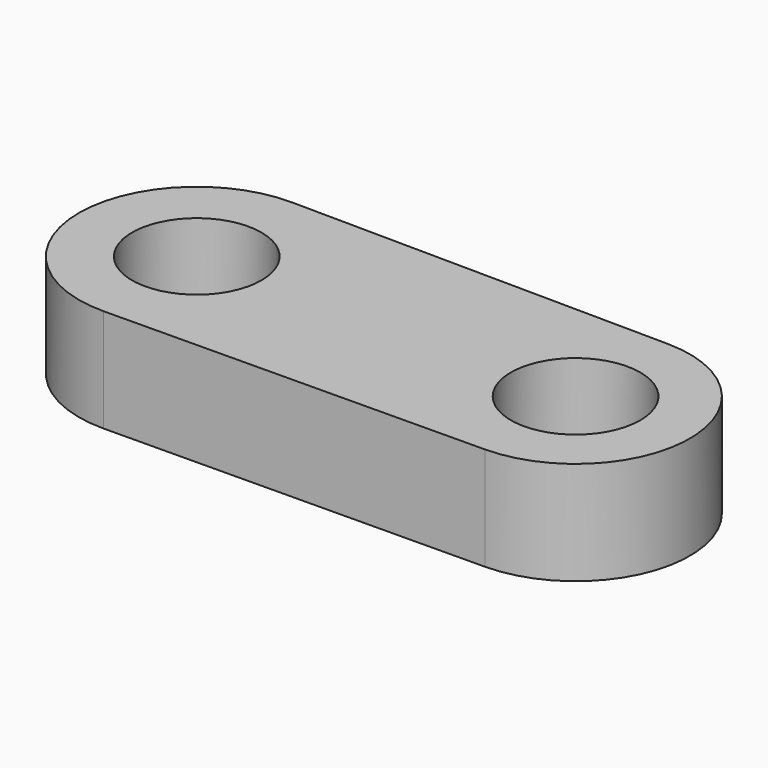
from build123d import *

# Parameters (mm, degrees)
F0_R     = 15.9206607186
F1_DEPTH = 25.4


# Not quite as in the source:
# - the program builds the solid bodies; features that only make, move or delete a surface that nothing else refers to are left out


with BuildPart() as f1:
    # F0 (on Top) → F1 (new body)
    with BuildSketch(Plane.XY):
        with BuildLine():
            ThreePointArc((-46.3083671537, -28.9735284728), (-17.6046094791, 0), (-46.3083671537, 28.9735284728))
            ThreePointArc((-46.3083671537, 28.9735284728), (-75.5542018517, 0), (-46.3083671537, -28.9735284728))
        make_face()
        with Locations((-46.5794056654, 0)):
            Circle(F0_R, mode=Mode.SUBTRACT)
        with BuildLine():
            Line((46.8422925338, 28.1021324953), (-46.3083671537, 28.9735284728))
            ThreePointArc((-46.3083671537, 28.9735284728), (-17.6046094791, 0), (-46.3083671537, -28.9735284728))
            Line((-46.3083671537, -28.9735284728), (46.8422925338, -28.1021324953))
            ThreePointArc((46.8422925338, -28.1021324953), (74.682767747, 0), (46.8422925338, 28.1021324953))
        make_face()
        with Locations((46.5794056654, 0)):
            Circle(F0_R, mode=Mode.SUBTRACT)
    extrude(amount=F1_DEPTH)


solid = f1.part
